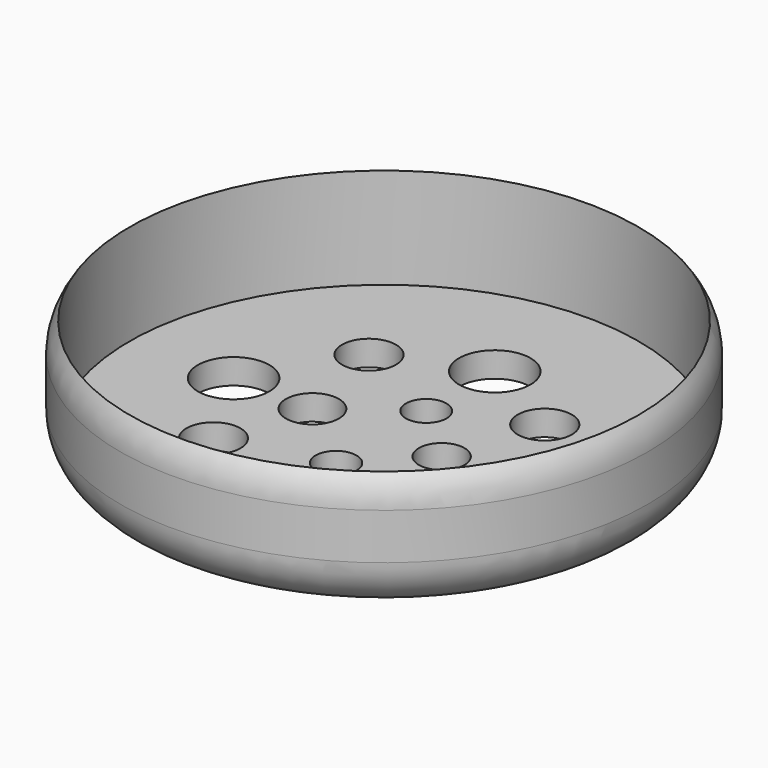
from build123d import *

# Parameters (mm, degrees)
F0_R     = 26.67
F0_R_2   = 25.7175
F1_DEPTH = 12.7
F0_R_3   = 3.6140603124
F0_R_4   = 2.7324582159
F0_R_5   = 2.6764413385
F0_R_6   = 2.0706768846
F0_R_7   = 2.3053611978
F0_R_8   = 2.0495959377
F2_DEPTH = 2.54
F3_R     = 5.08


# Not quite as in the source:
# - a fillet or chamfer that OpenCascade refuses, or shapes differently, is made with other operations: its cross-section is extruded or revolved along the edge and cut away or added


with BuildPart() as f1:
    # F0 (on Top) → F1 (new body)
    with BuildSketch(Plane.XY):
        Circle(F0_R)
        Circle(F0_R_2, mode=Mode.SUBTRACT)
    extrude(amount=F1_DEPTH)

    # F0 (on Top) → F2 (join)
    with BuildSketch(Plane.XY):
        Circle(F0_R_2)
        with Locations((-0.2498619724, -15.9751214087)):
            Circle(F0_R_3, mode=Mode.SUBTRACT)
        with Locations((-10.1906396449, -8.8177612051)):
            Circle(F0_R_4, mode=Mode.SUBTRACT)
        with Locations((-7.2378846817, 0)):
            Circle(F0_R_5, mode=Mode.SUBTRACT)
        with Locations((0, -6.0694427229)):
            Circle(F0_R_6, mode=Mode.SUBTRACT)
        with Locations((9.885732587, -8.9516246493)):
            Circle(F0_R_4, mode=Mode.SUBTRACT)
        with Locations((5.8176736347, 0)):
            Circle(F0_R_7, mode=Mode.SUBTRACT)
        with Locations((15.1746629134, -0.0083851115)):
            Circle(F0_R_3, mode=Mode.SUBTRACT)
        with Locations((-15.3598431498, 0.1952101447)):
            Circle(F0_R_3, mode=Mode.SUBTRACT)
        with Locations((0, 5.3194356151)):
            Circle(F0_R_8, mode=Mode.SUBTRACT)
        with Locations((-9.527919814, 10.0034438074)):
            Circle(F0_R_4, mode=Mode.SUBTRACT)
        with Locations((0, 13.979755342)):
            Circle(F0_R_3, mode=Mode.SUBTRACT)
        with Locations((8.7631102651, 9.3407258391)):
            Circle(F0_R_4, mode=Mode.SUBTRACT)
    extrude(amount=F2_DEPTH)

    # F3
    f3_edges = [f1.edges().sort_by_distance(p)[0] for p in [
        (-26.67, 0, 0),
    ]]
    fillet(f3_edges, radius=F3_R)

    # F4: fillet of radius 5.08 on 1 edges, made by hand

    # F4_s1 → F4_t2 (revolve, cut)
    with BuildSketch(Plane.XZ):
        with BuildLine():
            ThreePointArc((26.67, 9.7385571506), (26.4260159222, 11.2939831373), (25.7175, 12.7))
            Line((25.7175, 12.7), (26.67, 12.7))
            Line((26.67, 12.7), (26.67, 9.7385571506))
        make_face()
    revolve(axis=Axis((0, 0, 12.7), (0, 0, 1)), mode=Mode.SUBTRACT)


solid = f1.part
